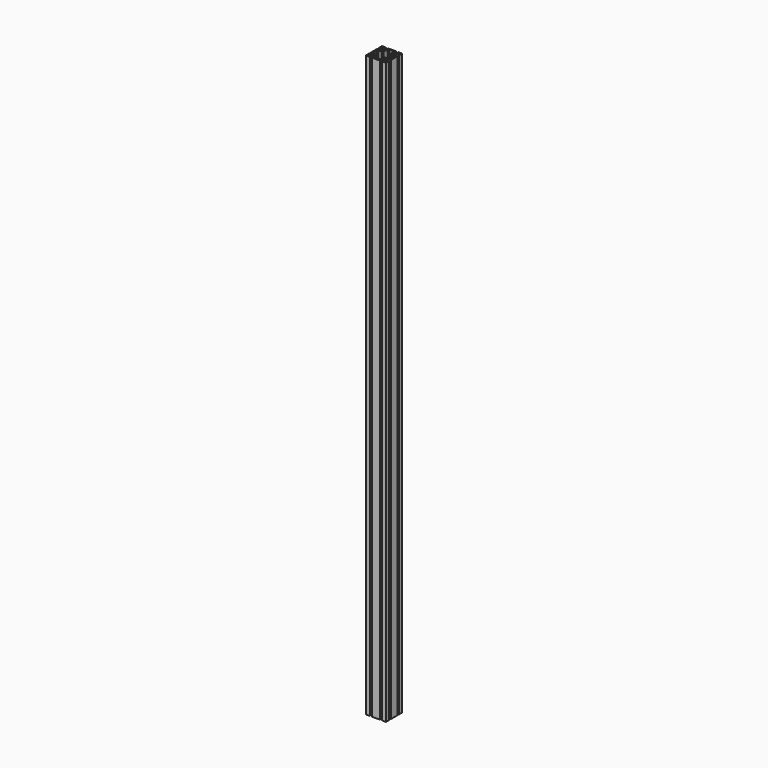
from build123d import *

# Parameters (mm, degrees)
F0_R     = 3
F0_R_2   = 2.5
F1_DEPTH = 1724
F2_R     = 2
F3_R     = 7


# Not quite as in the source:
# - a feature names something its author has since deleted; it is built from what else it names


with BuildPart() as f1:
    # F0 (on Top) → F1 (new body)
    with BuildSketch(Plane.XY):
        with BuildLine():
            Line((18.15, -30), (30, -30))
            Line((30, -30), (30, -18.15))
            Line((30, -18.15), (27.5, -18.15))
            Line((27.5, -18.15), (27.5, -20.15))
            Line((27.5, -20.15), (21.5477069044, -20.15))
            ThreePointArc((21.5477069044, -20.15), (19.5, -15), (21.5477069044, -9.85))
            Line((21.5477069044, -9.85), (27.5, -9.85))
            Line((27.5, -9.85), (27.5, -11.85))
            Line((27.5, -11.85), (30, -11.85))
            Line((30, -11.85), (30, 11.85))
            Line((30, 11.85), (27.5, 11.85))
            Line((27.5, 11.85), (27.5, 9.85))
            Line((27.5, 9.85), (21.5477069044, 9.85))
            ThreePointArc((21.5477069044, 9.85), (19.5, 15), (21.5477069044, 20.15))
            Line((21.5477069044, 20.15), (27.5, 20.15))
            Line((27.5, 20.15), (27.5, 18.15))
            Line((27.5, 18.15), (30, 18.15))
            Line((30, 18.15), (30, 30))
            Line((30, 30), (18.15, 30))
            Line((18.15, 30), (18.15, 27.5))
            Line((18.15, 27.5), (20.15, 27.5))
            Line((20.15, 27.5), (20.15, 21.5477069044))
            ThreePointArc((20.15, 21.5477069044), (15, 19.5), (9.85, 21.5477069044))
            Line((9.85, 21.5477069044), (9.85, 27.5))
            Line((9.85, 27.5), (11.85, 27.5))
            Line((11.85, 27.5), (11.85, 30))
            Line((11.85, 30), (-11.85, 30))
            Line((-11.85, 30), (-11.85, 27.5))
            Line((-11.85, 27.5), (-9.85, 27.5))
            Line((-9.85, 27.5), (-9.85, 21.5477069044))
            ThreePointArc((-9.85, 21.5477069044), (-15, 19.5), (-20.15, 21.5477069044))
            Line((-20.15, 21.5477069044), (-20.15, 27.5))
            Line((-20.15, 27.5), (-18.15, 27.5))
            Line((-18.15, 27.5), (-18.15, 30))
            Line((-18.15, 30), (-30, 30))
            Line((-30, 30), (-30, 18.15))
            Line((-30, 18.15), (-27.5, 18.15))
            Line((-27.5, 18.15), (-27.5, 20.15))
            Line((-27.5, 20.15), (-21.5477069044, 20.15))
            ThreePointArc((-21.5477069044, 20.15), (-19.5, 15), (-21.5477069044, 9.85))
            Line((-21.5477069044, 9.85), (-27.5, 9.85))
            Line((-27.5, 9.85), (-27.5, 11.85))
            Line((-27.5, 11.85), (-30, 11.85))
            Line((-30, 11.85), (-30, -11.85))
            Line((-30, -11.85), (-27.5, -11.85))
            Line((-27.5, -11.85), (-27.5, -9.85))
            Line((-27.5, -9.85), (-21.5477069044, -9.85))
            ThreePointArc((-21.5477069044, -9.85), (-19.5, -15), (-21.5477069044, -20.15))
            Line((-21.5477069044, -20.15), (-27.5, -20.15))
            Line((-27.5, -20.15), (-27.5, -18.15))
            Line((-27.5, -18.15), (-30, -18.15))
            Line((-30, -18.15), (-30, -30))
            Line((-30, -30), (-18.15, -30))
            Line((-18.15, -30), (-18.15, -27.5))
            Line((-18.15, -27.5), (-20.15, -27.5))
            Line((-20.15, -27.5), (-20.15, -21.5477069044))
            ThreePointArc((-20.15, -21.5477069044), (-15, -19.5), (-9.85, -21.5477069044))
            Line((-9.85, -21.5477069044), (-9.85, -27.5))
            Line((-9.85, -27.5), (-11.85, -27.5))
            Line((-11.85, -27.5), (-11.85, -30))
            Line((-11.85, -30), (11.85, -30))
            Line((11.85, -30), (11.85, -27.5))
            Line((11.85, -27.5), (9.85, -27.5))
            Line((9.85, -27.5), (9.85, -21.5477069044))
            ThreePointArc((9.85, -21.5477069044), (15, -19.5), (20.15, -21.5477069044))
            Line((20.15, -21.5477069044), (20.15, -27.5))
            Line((20.15, -27.5), (18.15, -27.5))
            Line((18.15, -27.5), (18.15, -30))
        make_face()
        with Locations((-25, -25)):
            Circle(F0_R, mode=Mode.SUBTRACT)
        with Locations((-15, -15)):
            Circle(F0_R_2, mode=Mode.SUBTRACT)
        with Locations((25, -25)):
            Circle(F0_R, mode=Mode.SUBTRACT)
        with Locations((15, -15)):
            Circle(F0_R_2, mode=Mode.SUBTRACT)
        with Locations((-25, 25)):
            Circle(F0_R, mode=Mode.SUBTRACT)
        with Locations((-15, 15)):
            Circle(F0_R_2, mode=Mode.SUBTRACT)
        Polygon((-7, 22), (-7, 27.5), (0, 27.5), (7, 27.5), (7, 22), (10, 16), (10, 10), (16, 10), (22, 7), (27.5, 7), (27.5, 0), (27.5, -7), (22, -7), (16, -10), (10, -10), (10, -16), (7, -22), (7, -27.5), (0, -27.5), (-7, -27.5), (-7, -22), (-10, -16), (-10, -10), (-16, -10), (-22, -7), (-27.5, -7), (-27.5, 0), (-27.5, 7), (-22, 7), (-16, 10), (-10, 10), (-10, 16), align=None, mode=Mode.SUBTRACT)
        with Locations((15, 15)):
            Circle(F0_R_2, mode=Mode.SUBTRACT)
        with Locations((25, 25)):
            Circle(F0_R, mode=Mode.SUBTRACT)
    extrude(amount=F1_DEPTH)

    # F2
    f2_edges = [f1.edges().sort_by_distance(p)[0] for p in [
        (-7, 27.5, 862),
        (7, 27.5, 862),
    ]]
    fillet(f2_edges, radius=F2_R)

    # F3
    f3_edges = [f1.edges().sort_by_distance(p)[0] for p in [
        (-10, 16, 862),
        (10, 16, 862),
    ]]
    fillet(f3_edges, radius=F3_R)


solid = f1.part
